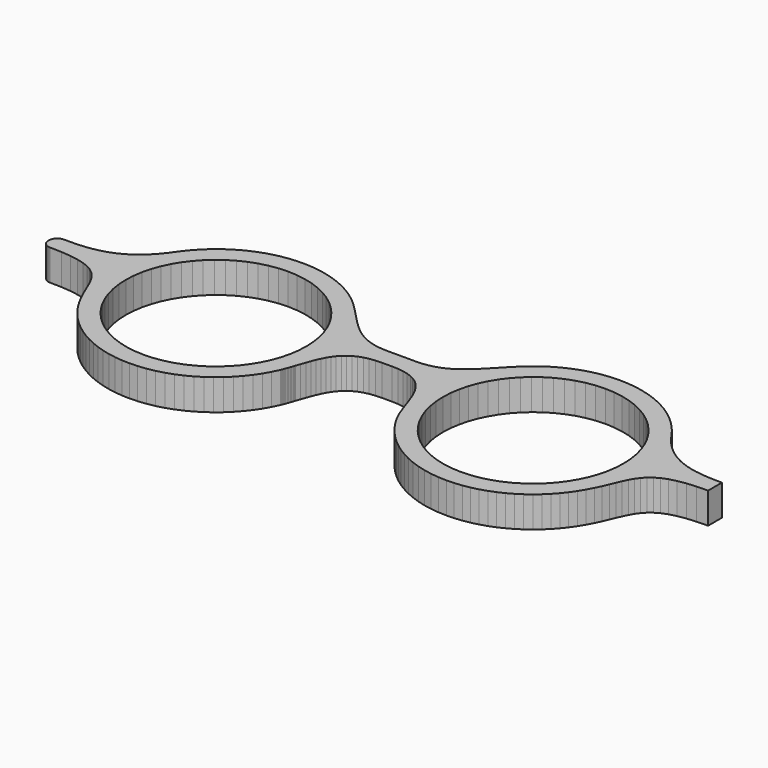
from build123d import *

# Parameters (mm, degrees)
F1_DEPTH = 6


with BuildPart() as f1:
    # F0 (on Top) → F1 (new body)
    with BuildSketch(Plane.XY):
        Polygon((48.825615, 11.996856), (48.832506, 11.986521), (48.83285, 11.986521), (48.832161, 11.988071), (48.830783, 11.990483), (48.828716, 11.993755), (48.82596, 11.997545), (48.823204, 12.001679), (48.820792, 12.005469), (48.818381, 12.008914), (48.816314, 12.01167), (48.81528, 12.013392), (48.814591, 12.013737), (48.81528, 12.012703), (48.817347, 12.009603), (48.820448, 12.004435), align=None)
    extrude(amount=F1_DEPTH)


with BuildPart() as f1b:
    # F0 (on Top) → F1, piece 2 (new body)
    with BuildSketch(Plane.XY):
        Polygon((-46.415772, 12.986287), (-47.157501, 11.986521), (-47.96951, 10.853429), (-48.796677, 9.838331), (-49.63797, 8.934855), (-50.49287, 8.136799), (-51.36069, 7.437789), (-52.240395, 6.831452), (-53.131641, 6.311587), (-54.033567, 5.871821), (-54.945311, 5.505952), (-55.866358, 5.207434), (-56.795845, 4.970067), (-57.733083, 4.787477), (-58.677211, 4.653463), (-59.627713, 4.561479), (-60.583727, 4.505496), (-61.544564, 4.478969), (-61.631725, 4.478452), (-61.719058, 4.477935), (-61.806391, 4.477418), (-61.893552, 4.476902), (-61.980713, 4.476385), (-62.068046, 4.475868), (-62.15538, 4.475179), (-62.242541, 4.474662), (-62.329701, 4.474145), (-62.417035, 4.473456), (-62.504368, 4.47294), (-62.591529, 4.472423), (-62.67869, 4.471906), (-62.766023, 4.471389), (-62.853356, 4.470873), (-62.940517, 4.470356), (-62.940517, 4.470184), (-62.940517, 4.470011), (-62.940517, 4.469839), (-62.940517, 4.469667), (-62.940517, 4.469495), (-62.940517, 4.469322), (-63.111738, 4.46071), (-63.278136, 4.435216), (-63.438678, 4.394047), (-63.592501, 4.33772), (-63.738918, 4.267267), (-63.877066, 4.183379), (-64.005913, 4.086917), (-64.124941, 3.978741), (-64.233117, 3.859713), (-64.329579, 3.730866), (-64.413467, 3.592718), (-64.48392, 3.446301), (-64.540247, 3.292478), (-64.581416, 3.131936), (-64.60691, 2.965538), (-64.615522, 2.794317), (-64.60691, 2.623096), (-64.581416, 2.456698), (-64.540247, 2.296156), (-64.48392, 2.142333), (-64.413467, 1.995916), (-64.329579, 1.857768), (-64.233117, 1.728921), (-64.124941, 1.609893), (-64.005913, 1.501717), (-63.877066, 1.405254), (-63.738918, 1.321366), (-63.592501, 1.250914), (-63.438678, 1.194587), (-63.278136, 1.153418), (-63.111738, 1.127924), (-62.940517, 1.119311), (-62.940517, 1.119139), (-62.940517, 1.118967), (-62.940517, 1.118795), (-62.940517, 1.118622), (-62.940517, 1.11845), (-62.940517, 1.118278), (-60.757877, 1.064362), (-58.879094, 0.905371), (-57.275402, 0.645266), (-55.917517, 0.287665), (-54.776846, -0.162953), (-53.82445, -0.703144), (-53.031389, -1.328773), (-52.368897, -2.035707), (-51.808035, -2.820155), (-51.320038, -3.678329), (-50.875792, -4.606437), (-50.446534, -5.600347), (-50.003494, -6.655925), (-49.517736, -7.769379), (-48.960147, -8.936922), (-48.301962, -10.154075), (-47.591238, -11.342288), (-46.806273, -12.478136), (-45.950512, -13.558518), (-45.027398, -14.579989), (-44.039862, -15.539448), (-42.991864, -16.433106), (-41.886333, -17.257517), (-40.726886, -18.009926), (-39.516796, -18.686198), (-38.259508, -19.283233), (-36.958296, -19.79793), (-35.616603, -20.2265), (-34.237704, -20.565842), (-32.825215, -20.812166), (-31.382064, -20.962717), (-29.912386, -21.013704), (-28.314896, -20.95376), (-26.749789, -20.775993), (-25.221544, -20.485571), (-23.734297, -20.086629), (-22.29218, -19.583301), (-20.899672, -18.980065), (-19.561253, -18.281055), (-18.281055, -17.491094), (-17.063558, -16.613973), (-15.913241, -15.654514), (-14.834237, -14.617196), (-13.830681, -13.505808), (-12.907051, -12.324829), (-12.06817, -11.079083), (-11.317828, -9.772358), (-10.660504, -8.409478), (-10.652925, -8.390875), (-10.63191, -8.33782), (-10.598837, -8.253415), (-10.554739, -8.141794), (-10.50134, -8.006057), (-10.440707, -7.849995), (-10.374216, -7.677051), (-10.303247, -7.490671), (-10.229178, -7.29499), (-10.154075, -7.092763), (-10.078972, -6.888468), (-10.005936, -6.684863), (-9.936, -6.486081), (-9.871232, -6.295223), (-9.812666, -6.115734), (-9.762367, -5.951747), (-9.455065, -5.053266), (-9.149829, -4.177178), (-8.838048, -3.327962), (-8.510764, -2.510441), (-8.159365, -1.729783), (-7.774547, -0.991154), (-7.3477, -0.299034), (-6.87021, 0.341409), (-6.333464, 0.925008), (-5.727816, 1.447112), (-5.044998, 1.902382), (-4.276053, 2.285993), (-3.412023, 2.592951), (-2.44464, 2.818433), (-1.364603, 2.95727), (-0.162609, 3.004812), (-0.037552, 3.004812), (0.087505, 3.004812), (0.212562, 3.004812), (0.337619, 3.004812), (0.462676, 3.004812), (0.587733, 3.004812), (0.712445, 3.004812), (0.837502, 3.004812), (0.962559, 3.004812), (1.087272, 3.004812), (1.212329, 3.004812), (1.337386, 3.004812), (1.462443, 3.004812), (1.5875, 3.004812), (1.712557, 3.004812), (1.837614, 3.004812), (3.039607, 2.95727), (4.119645, 2.818433), (5.087028, 2.592951), (5.951058, 2.285993), (6.720003, 1.902382), (7.402821, 1.447112), (8.008469, 0.925008), (8.545214, 0.341409), (9.022705, -0.299034), (9.449552, -0.991154), (9.834369, -1.729783), (10.185769, -2.510441), (10.513053, -3.327962), (10.824834, -4.177178), (11.13007, -5.053266), (11.437372, -5.951747), (11.493527, -6.105054), (11.549338, -6.258705), (11.605493, -6.412356), (11.661648, -6.566008), (11.717803, -6.719659), (11.773958, -6.87331), (11.830113, -7.026961), (11.886268, -7.180613), (11.942423, -7.334264), (11.998578, -7.487915), (12.054733, -7.641566), (12.110888, -7.795218), (12.167043, -7.948869), (12.223198, -8.10252), (12.279353, -8.256171), (12.335509, -8.409478), (12.992833, -9.772358), (13.743175, -11.079083), (14.582055, -12.324829), (15.505685, -13.505808), (16.509242, -14.617196), (17.588246, -15.654514), (18.738563, -16.613973), (19.95606, -17.491094), (21.236257, -18.281055), (22.574677, -18.980065), (23.967184, -19.583301), (25.409301, -20.086629), (26.896549, -20.485571), (28.424793, -20.775993), (29.9899, -20.95376), (31.587391, -21.013704), (33.057069, -20.963062), (34.500219, -20.812855), (35.912708, -20.566531), (37.29178, -20.227878), (38.6333, -19.799653), (39.934513, -19.285645), (41.191628, -18.689299), (42.401546, -18.013715), (43.56082, -17.26234), (44.666352, -16.438273), (45.71435, -15.545304), (46.70137, -14.586534), (47.624311, -13.565408), (48.480417, -12.485371), (49.265554, -11.349523), (49.975933, -10.161654), (50.633946, -8.944157), (51.191707, -7.776614), (51.677465, -6.66247), (52.120849, -5.606548), (52.550108, -4.612294), (52.994525, -3.683496), (53.482695, -2.824634), (54.043557, -2.039497), (54.706049, -1.331529), (55.49911, -0.705556), (56.451679, -0.164676), (57.59235, 0.286632), (58.950407, 0.644577), (60.554098, 0.905027), (62.433054, 1.064362), (64.615522, 1.118278), (64.615522, 1.491382), (64.615522, 1.800924), (64.615522, 2.055861), (64.615522, 2.264978), (64.615522, 2.437405), (64.615522, 2.581927), (64.615522, 2.707673), (64.615522, 2.8236), (64.615522, 2.938494), (64.615522, 3.061484), (64.615522, 3.201527), (64.615522, 3.367409), (64.615522, 3.56843), (64.615522, 3.813204), (64.615522, 4.11086), (64.615522, 4.470356), (63.553743, 4.478452), (62.498166, 4.508596), (61.450168, 4.569058), (60.410782, 4.668449), (59.379665, 4.81521), (58.358539, 5.017954), (57.347404, 5.285121), (56.347292, 5.62498), (55.359239, 6.046143), (54.383243, 6.557395), (53.421028, 7.166832), (52.472249, 7.88324), (51.538628, 8.714886), (50.620166, 9.670383), (49.717895, 10.758), (48.832506, 11.986521), (48.091121, 12.986287), (47.293237, 13.939373), (46.441265, 14.843711), (45.537961, 15.696544), (44.585736, 16.495462), (43.587003, 17.238224), (42.544173, 17.922076), (41.460001, 18.54426), (40.336556, 19.10271), (39.176936, 19.59467), (37.982866, 20.017899), (36.757101, 20.369816), (35.502398, 20.647663), (34.220822, 20.849373), (32.915131, 20.972191), (31.587391, 21.013704), (30.498396, 20.985799), (29.423527, 20.902945), (28.36416, 20.766691), (27.322018, 20.578244), (26.297792, 20.338982), (25.293546, 20.050456), (24.310316, 19.713698), (23.349479, 19.330431), (22.412757, 18.901861), (21.500841, 18.429538), (20.615451, 17.914496), (19.758311, 17.358458), (18.93011, 16.762457), (18.132571, 16.128214), (17.36707, 15.456765), (16.634988, 14.749832), (15.849506, 13.966934), (15.099164, 13.193682), (14.37535, 12.435417), (13.669794, 11.697994), (12.974229, 10.987098), (12.280387, 10.308242), (11.579655, 9.667282), (10.863764, 9.069731), (10.124446, 8.521271), (9.353434, 8.027589), (8.542458, 7.594368), (7.682907, 7.227293), (6.766167, 6.931877), (5.784659, 6.713802), (4.729427, 6.578754), (3.592201, 6.53259), (3.248036, 6.53259), (2.903526, 6.53259), (2.559017, 6.53259), (2.214852, 6.53259), (1.870686, 6.53259), (1.526177, 6.53259), (1.181667, 6.53259), (0.837502, 6.53259), (0.493337, 6.53259), (0.148828, 6.53259), (-0.195682, 6.53259), (-0.539847, 6.53259), (-0.884012, 6.53259), (-1.228521, 6.53259), (-1.573031, 6.53259), (-1.917196, 6.53259), (-3.054422, 6.578754), (-4.109655, 6.713802), (-5.091162, 6.931877), (-6.007902, 7.227293), (-6.867454, 7.594368), (-7.678429, 8.027589), (-8.449442, 8.521271), (-9.188759, 9.069731), (-9.90465, 9.667282), (-10.605382, 10.308242), (-11.299225, 10.987098), (-11.994789, 11.697994), (-12.700345, 12.435417), (-13.424159, 13.193682), (-14.174501, 13.966934), (-14.959983, 14.749832), (-15.692066, 15.456765), (-16.457566, 16.128214), (-17.255106, 16.762457), (-18.083307, 17.358458), (-18.940446, 17.914496), (-19.825836, 18.429538), (-20.737753, 18.901861), (-21.674474, 19.330431), (-22.635311, 19.713698), (-23.618541, 20.050456), (-24.622787, 20.338982), (-25.647014, 20.578244), (-26.689155, 20.766691), (-27.748522, 20.902945), (-28.823392, 20.985799), (-29.912386, 21.013704), (-31.240126, 20.972191), (-32.545817, 20.849373), (-33.827221, 20.647663), (-35.082097, 20.369816), (-36.307689, 20.017899), (-37.50176, 19.59467), (-38.661723, 19.10271), (-39.784997, 18.54426), (-40.86934, 17.922076), (-41.911999, 17.238224), (-42.910732, 16.495462), (-43.862956, 15.696544), (-44.766088, 14.843711), (-45.617888, 13.939373), align=None)
        Polygon((-12.42646, 0), (-12.517066, -1.785249), (-12.782338, -3.51951), (-13.214009, -5.194171), (-13.802775, -6.79993), (-14.540026, -8.328174), (-15.416803, -9.769946), (-16.424493, -11.11629), (-17.553795, -12.358591), (-18.796097, -13.487893), (-20.14244, -14.495584), (-21.584213, -15.372361), (-23.112457, -16.109611), (-24.718216, -16.698378), (-26.392532, -17.130048), (-28.127138, -17.395321), (-29.912386, -17.485927), (-31.697635, -17.395321), (-33.432068, -17.130048), (-35.106557, -16.698378), (-36.712144, -16.109611), (-38.240388, -15.372361), (-39.68216, -14.495584), (-41.028676, -13.487893), (-42.270977, -12.358591), (-43.400452, -11.11629), (-44.40797, -9.769946), (-45.284747, -8.328174), (-46.021997, -6.79993), (-46.610937, -5.194171), (-47.042435, -3.51951), (-47.307879, -1.785249), (-47.398313, 0), (-47.307879, 1.785248), (-47.042435, 3.519509), (-46.610937, 5.193826), (-46.021997, 6.799585), (-45.284747, 8.327657), (-44.40797, 9.769429), (-43.400452, 11.115945), (-42.270977, 12.358246), (-41.028676, 13.487721), (-39.68216, 14.495239), (-38.240388, 15.372016), (-36.712144, 16.109266), (-35.106557, 16.698205), (-33.432068, 17.129704), (-31.697635, 17.395148), (-29.912386, 17.485582), (-28.127138, 17.395148), (-26.392532, 17.129704), (-24.718216, 16.698205), (-23.112457, 16.109266), (-21.584213, 15.372016), (-20.14244, 14.495239), (-18.796097, 13.487721), (-17.553795, 12.358246), (-16.424493, 11.115945), (-15.416803, 9.769429), (-14.540026, 8.327657), (-13.802775, 6.799585), (-13.214009, 5.193826), (-12.782338, 3.519509), (-12.517066, 1.785248), align=None, mode=Mode.SUBTRACT)
        Polygon((49.073318, 0), (48.982712, -1.785249), (48.717439, -3.51951), (48.285769, -5.194171), (47.697002, -6.79993), (46.959752, -8.328174), (46.082975, -9.769946), (45.075284, -11.11629), (43.945982, -12.358591), (42.703681, -13.487893), (41.357337, -14.495584), (39.915565, -15.372361), (38.387321, -16.109611), (36.781562, -16.698378), (35.107245, -17.130048), (33.37264, -17.395321), (31.587391, -17.485927), (29.802143, -17.395321), (28.067537, -17.130048), (26.393221, -16.698378), (24.787462, -16.109611), (23.259217, -15.372361), (21.817445, -14.495584), (20.471102, -13.487893), (19.2288, -12.358591), (18.099498, -11.11629), (17.091807, -9.769946), (16.215031, -8.328174), (15.47778, -6.79993), (14.889013, -5.194171), (14.457343, -3.51951), (14.19207, -1.785249), (14.101464, 0), (14.19207, 1.785248), (14.457343, 3.519509), (14.889013, 5.193826), (15.47778, 6.799585), (16.215031, 8.327657), (17.091807, 9.769429), (18.099498, 11.115945), (19.2288, 12.358246), (20.471102, 13.487721), (21.817445, 14.495239), (23.259217, 15.372016), (24.787462, 16.109266), (26.393221, 16.698205), (28.067537, 17.129704), (29.802143, 17.395148), (31.587391, 17.485582), (33.37264, 17.395148), (35.107245, 17.129704), (36.781562, 16.698205), (38.387321, 16.109266), (39.915565, 15.372016), (41.357337, 14.495239), (42.703681, 13.487721), (43.945982, 12.358246), (45.075284, 11.115945), (46.082975, 9.769429), (46.959752, 8.327657), (47.697002, 6.799585), (48.285769, 5.193826), (48.717439, 3.519509), (48.982712, 1.785248), align=None, mode=Mode.SUBTRACT)
    extrude(amount=F1_DEPTH)


solid = Compound([f1.part, f1b.part])
